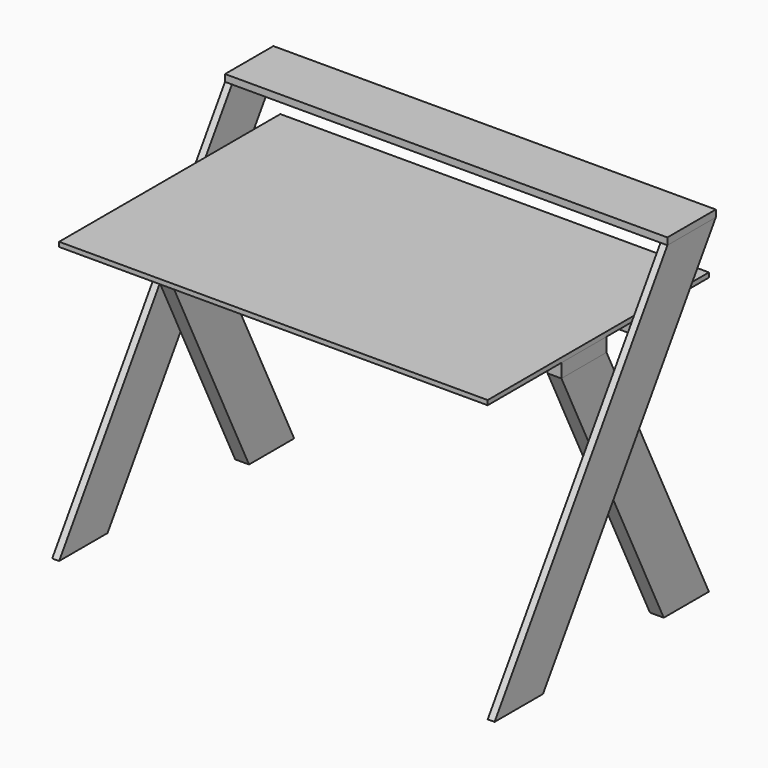
from build123d import *

# Parameters (mm, degrees)
F0_W      = 19.05
F0_H      = 762
F1_DEPTH  = 914.4
F3_DEPTH  = 1219.201
F4_W      = 1219.2
F4_H      = 166.6968156723
F5_DEPTH  = 19.05
F7_DEPTH  = 38.1
F8_W      = 38.1
F8_H      = 155.3915016532
F9_DEPTH  = 38.1
F8_W_2    = 1181.1
F8_H_2    = 88.9
F11_W     = 762
F11_H     = 12.7
F12_DEPTH = 1181.1


with BuildPart() as f1:
    # F0 (on Top) → F1 (new body)
    with BuildSketch(Plane.XY):
        with Locations((-600.075, 0)):
            Rectangle(F0_W, F0_H)
    extrude(amount=F1_DEPTH)


with BuildPart() as f1b:
    # F0 (on Top) → F1, piece 2 (new body)
    with BuildSketch(Plane.XY):
        with Locations((600.075, 0)):
            Rectangle(F0_W, F0_H)
    extrude(amount=F1_DEPTH)


with BuildPart() as f3_tool:
    # F2 (on face) → F3 (new body, through all)
    with BuildSketch(Plane.YZ.offset(609.6)):
        Polygon((381, 914.4), (-214.3031843277, 0), (381, 0), align=None)
        Polygon((-381, 0), (214.3031843277, 914.4), (-381, 914.4), align=None)
    extrude(amount=-F3_DEPTH)


with BuildPart() as f1_1:
    add(f1.part)

    # F3: cut by f3_tool
    add(f3_tool.part, mode=Mode.SUBTRACT)


with BuildPart() as f1b_1:
    add(f1b.part)

    # F3: cut by f3_tool
    add(f3_tool.part, mode=Mode.SUBTRACT)


with BuildPart() as f5:
    # F4 (on face) → F5 (new body)
    with BuildSketch(Plane.XY.offset(914.4)):
        with Locations((0, 297.6515921639)):
            Rectangle(F4_W, F4_H)
    extrude(amount=F5_DEPTH)


with BuildPart() as f7:
    # F6 (on face) → F7 (new body)
    with BuildSketch(Plane.YZ.offset(-590.55)):
        Polygon((225.6084983468, 0), (381, 0), (28.3915016532, 723.9), (-127, 723.9), align=None)
    extrude(amount=F7_DEPTH)


with BuildPart() as f9:
    # F8 (on face) → F9 (new body)
    with BuildSketch(Plane.XY.offset(723.9)):
        with Locations((-571.5, -49.3042491734)):
            Rectangle(F8_W, F8_H)
    extrude(amount=F9_DEPTH)


with BuildPart() as f9b:
    # F8 (on face) → F9, piece 2 (new body)
    with BuildSketch(Plane.XY.offset(723.9)):
        with Locations((0, 173.6300954289)):
            Rectangle(F8_W_2, F8_H_2)
    extrude(amount=F9_DEPTH)


with BuildPart() as f10_1:
    # F10: instance of F7
    add(f7.part.mirror(Plane.YZ))


with BuildPart() as f10_2:
    # F10: instance of F9
    add(f9.part.mirror(Plane.YZ))


with BuildPart() as f12:
    # F11 (on face) → F12 (new body, through all)
    with BuildSketch(Plane.YZ.offset(-590.55)):
        with Locations((0, 768.35)):
            Rectangle(F11_W, F11_H)
    extrude(amount=F12_DEPTH)


solid = Compound([f1_1.part, f1b_1.part, f5.part, f7.part, f9.part, f9b.part, f10_1.part, f10_2.part, f12.part])
